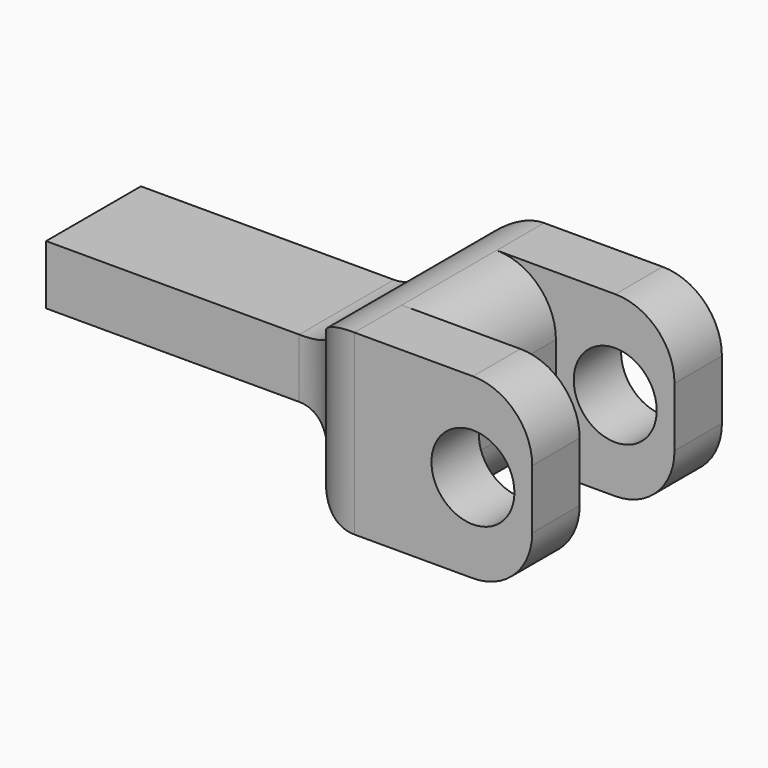
from build123d import *

# Parameters (mm, degrees)
F1_DEPTH = 7.5
F3_D     = 7
F4_R     = 5
F5_R     = 4.99999
F6_W     = 10
F6_H     = 5
F7_DEPTH = 25
F8_R     = 5


# Not quite as in the source:
# - a fillet or chamfer is up to 0.001 mm smaller than in the source, because OpenCascade refuses the exact size


with BuildPart() as f1:
    # F0 (on Top) → F1 (new body, symmetric)
    with BuildSketch(Plane.XY):
        Polygon((10, 10), (-10, 10), (-10, -10), (10, -10), (10, -5), (0, -5), (0, 5), (10, 5), align=None)
    extrude(amount=F1_DEPTH, both=True)

    # F3 (through all)
    with Locations(Plane(origin=(0, 10, 0), x_dir=(-1, 0, 0), z_dir=(0, 1, 0))):
        with Locations((-5, 0)):
            Hole(F3_D / 2)

    # F4
    f4_edges = [f1.edges().sort_by_distance(p)[0] for p in [
        (10, 7.5, 7.5),
        (10, 7.5, -7.5),
        (10, -7.5, 7.5),
        (10, -7.5, -7.5),
        (-10, 10, 0),
        (-10, 0, -7.5),
        (-10, -10, 0),
        (-10, 0, 7.5),
    ]]
    fillet(f4_edges, radius=F4_R)

    # F5 (radius 5 in the source; OpenCascade refuses exactly that, so slightly less here)
    f5_edges = [f1.edges().sort_by_distance(p)[0] for p in [
        (0, 0, 7.5),
        (0, 0, -7.5),
    ]]
    fillet(f5_edges, radius=F5_R)

    # F6 (on face) → F7 (join)
    with BuildSketch(Plane(origin=(-10, 0, 0), x_dir=(0, -1, 0), z_dir=(-1, 0, 0))):
        Rectangle(F6_W, F6_H)
    extrude(amount=F7_DEPTH)

    # F8
    f8_edges = [f1.edges().sort_by_distance(p)[0] for p in [
        (-10, 0, 2.5),
        (-10, -5, 0),
        (-10, 0, -2.5),
        (-10, 5, 0),
    ]]
    fillet(f8_edges, radius=F8_R)


solid = f1.part
